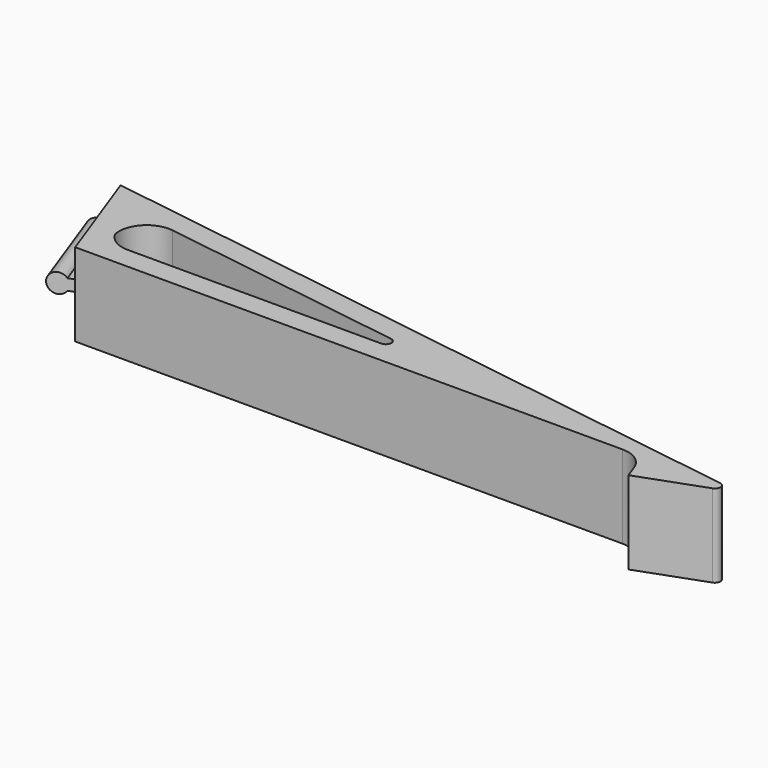
from build123d import *

# Parameters (mm, degrees)
F1_DEPTH    = 15
F2_T1_DEPTH = 15
F3_R        = 1
F6_DEPTH    = 17.5


# Not quite as in the source:
# - a fillet or chamfer that OpenCascade refuses, or shapes differently, is made with other operations: its cross-section is extruded or revolved along the edge and cut away or added


with BuildPart() as f1:
    # F0 (on Top) → F1 (new body)
    with BuildSketch(Plane.XY):
        Polygon((-63.4202014333, 5.036846236), (-56.5797985667, -13.7570061798), (45.8773750323, -13.7570061798), (63.4202014333, -13.7570061798), align=None)
        Polygon((-57.3651718984, 0.0960069154), (9.1331767526, -9.7570061798), (-53.7789684139, -9.7570061798), align=None, mode=Mode.SUBTRACT)
        Polygon((63.4202014333, -13.7570061798), (45.8773750323, -13.7570061798), (47.9294958922, -19.3951619045), align=None)
    extrude(amount=F1_DEPTH)

    # F2: fillet of radius 5 on 3 edges, made by hand

    # F2_s2 → F2_t1 (join)
    with BuildSketch(Plane.XY):
        with BuildLine():
            ThreePointArc((42.3763373412, -13.7570061798), (45.244219523, -14.6612459583), (47.0748004452, -17.0469054631))
            Line((47.0748004452, -17.0469054631), (45.8773750323, -13.7570061798))
            Line((45.8773750323, -13.7570061798), (42.3763373412, -13.7570061798))
        make_face()
        with BuildLine():
            ThreePointArc((-50.2779307229, -9.7570061798), (-53.1458129046, -8.8527664012), (-54.9763938268, -6.4671068964))
            Line((-54.9763938268, -6.4671068964), (-53.7789684139, -9.7570061798))
            Line((-53.7789684139, -9.7570061798), (-50.2779307229, -9.7570061798))
        make_face()
        with BuildLine():
            ThreePointArc((-49.0635393533, -1.1340400833), (-53.6703308808, -2.9189438256), (-54.4948480837, -7.790142952))
            Line((-54.4948480837, -7.790142952), (-57.3651718984, 0.0960069154))
            Line((-57.3651718984, 0.0960069154), (-49.0635393533, -1.1340400833))
        make_face()
    extrude(amount=F2_T1_DEPTH)

    # F3
    f3_edges = [f1.edges().sort_by_distance(p)[0] for p in [
        (63.420201, -13.757006, 7.5),
        (9.133177, -9.757006, 7.5),
    ]]
    fillet(f3_edges, radius=F3_R)

    # F5 (on face) → F6 (join)
    with BuildSketch(Plane(origin=(-9.0375654481, 24.8305069955, 0), x_dir=(-0.9396926208, -0.3420201433, 0), z_dir=(-0.3420201433, 0.9396926208, 0))):
        with BuildLine():
            Line((57.8727924241, 8.5), (57.8727924241, 6.5))
            Line((57.8727924241, 6.5), (59.8727924241, 6.5))
            ThreePointArc((59.8727924241, 6.5), (63.0589330857, 7.5), (59.8727924241, 8.5))
            Line((59.8727924241, 8.5), (57.8727924241, 8.5))
        make_face()
    extrude(amount=-F6_DEPTH)


solid = f1.part
